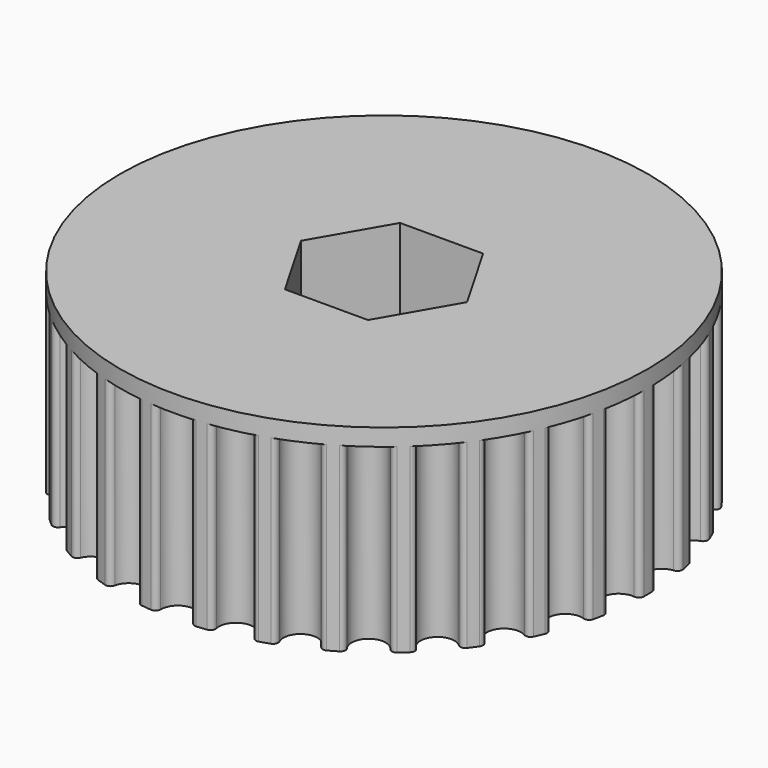
from build123d import *

# Parameters (mm, degrees)
F2_R            = 23.3007414911
F3_DEPTH        = 16
F5_DEPTH        = 16
F5_COPIES_COUNT = 30
F7_R            = 23.3007414911
F8_DEPTH        = 1.5
F10_DEPTH       = 17.501


# Not quite as in the source:
# - a feature of the source that left no trace in its solid (it failed there, or was rolled back) is left out
# - a pattern or mirror of a feature is missing from the dataset's text; its kind, count and spacing are read off the source's solid


with BuildPart() as f3:
    # F2 (on Top) → F3 (new body)
    with BuildSketch(Plane.XY):
        Circle(F2_R)
    extrude(amount=F3_DEPTH)

    # F4 (on face) → F5 (cut, through all)
    with BuildSketch(Plane.XY.offset(16)):
        with BuildLine():
            ThreePointArc((-1.9882155288, 23.2157608758), (-1.6432389463, 23.0968097974), (-1.4998597988, 22.7612496365))
            ThreePointArc((-1.4998597988, 22.7612496365), (0, 21.2407414911), (1.4998597988, 22.7612496365))
            ThreePointArc((1.4998597988, 22.7612496365), (1.6432389463, 23.0968097974), (1.9882155288, 23.2157608758))
            ThreePointArc((1.9882155288, 23.2157608758), (0, 23.3007414911), (-1.9882155288, 23.2157608758))
        make_face()
    f5 = extrude(amount=-F5_DEPTH, mode=Mode.SUBTRACT)

    # F5_copies: F5 ×30 about axis
    f5_copies_axis = Axis((0, 0, 0), (0, 0, 1))
    for i in range(1, F5_COPIES_COUNT):
        add(f5.rotate(f5_copies_axis, i * 360 / F5_COPIES_COUNT), mode=Mode.SUBTRACT)

    # F7 (on face) → F8 (join)
    with BuildSketch(Plane.XY.offset(16)):
        Circle(F7_R)
    extrude(amount=F8_DEPTH)

    # F9 (on face) → F10 (cut, through all)
    with BuildSketch(Plane.XY.offset(17.5)):
        Polygon((-3.6661742094, -6.35), (3.6661742094, -6.35), (7.3323484187, 0), (3.6661742094, 6.35), (-3.6661742094, 6.35), (-7.3323484187, 0), align=None)
    extrude(amount=-F10_DEPTH, mode=Mode.SUBTRACT)


solid = f3.part
